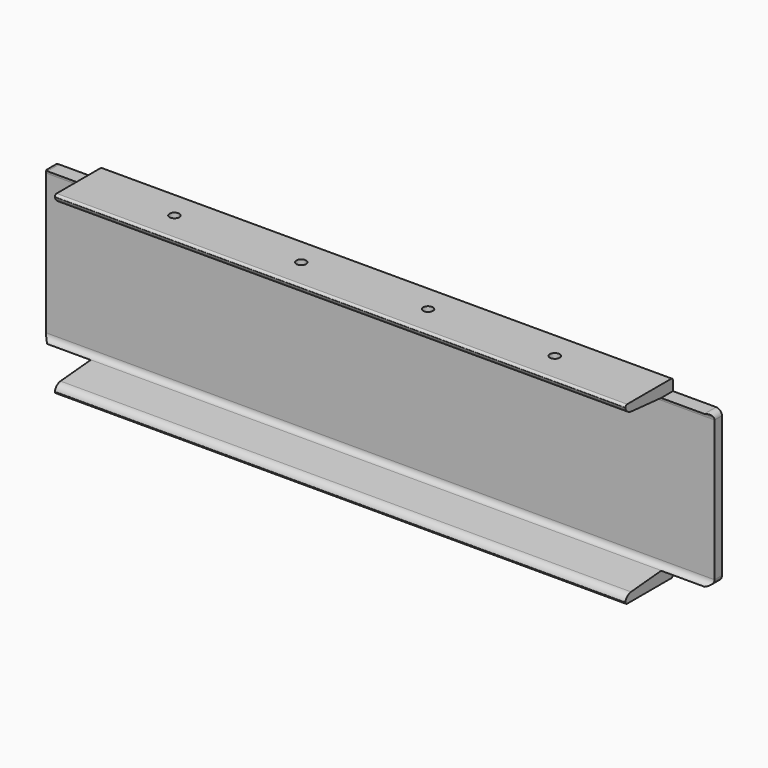
from build123d import *

# Parameters (mm, degrees)
F1_DEPTH    = 290
F2_T1_DEPTH = 611.1034588044
F3_R        = 4.25
F4_DEPTH    = 25
F5_W        = 60
F5_H        = 130.8605410159
F6_DEPTH    = 10.2
F7_R        = 5


# Not quite as in the source:
# - a fillet or chamfer that OpenCascade refuses, or shapes differently, is made with other operations: its cross-section is extruded or revolved along the edge and cut away or added
# - a pattern or mirror of a feature is missing from the dataset's text; its kind, count and spacing are read off the source's solid


with BuildPart() as f1:
    # F0 (on Right) → F1 (new body, symmetric)
    with BuildSketch(Plane.YZ):
        with BuildLine():
            ThreePointArc((-25.83, -74.2), (-25.2442135624, -75.6142135624), (-23.83, -76.2))
            Line((-23.83, -76.2), (23.83, -76.2))
            ThreePointArc((23.83, -76.2), (25.2442135624, -75.6142135624), (25.83, -74.2))
            Line((25.83, -74.2), (25.83, 74.2))
            ThreePointArc((25.83, 74.2), (25.2442135624, 75.6142135624), (23.83, 76.2))
            Line((23.83, 76.2), (-23.83, 76.2))
            ThreePointArc((-23.83, 76.2), (-25.2442135624, 75.6142135624), (-25.83, 74.2))
            Line((-25.83, 74.2), (-25.83, 69.4007524114))
            Line((-25.83, 69.4007524114), (13.2857787137, 65.978565209))
            ThreePointArc((13.2857787137, 65.978565209), (16.5363866841, 64.3755427566), (17.85, 60.9975917185))
            Line((17.85, 60.9975917185), (17.85, -60.9975917185))
            ThreePointArc((17.85, -60.9975917185), (16.5363866841, -64.3755427566), (13.2857787137, -65.978565209))
            Line((13.2857787137, -65.978565209), (-25.83, -69.4007524114))
            Line((-25.83, -69.4007524114), (-25.83, -74.2))
        make_face()
    extrude(amount=F1_DEPTH, both=True)

    # F2: fillet of radius 7 on 2 edges, made by hand

    # F2_s2 → F2_t1 (cut)
    with BuildSketch(Plane.YZ.offset(-305.5517294022)):
        with BuildLine():
            ThreePointArc((-25.83, -74.2), (-23.5930536317, -70.5297202282), (-19.6329798493, -68.8585834006))
            Line((-19.6329798493, -68.8585834006), (-19.6451816533, -68.7191161428))
            Line((-19.6451816533, -68.7191161428), (-25.842201804, -69.2612851537))
            Line((-25.842201804, -69.2612851537), (-25.97, -69.4007524114))
            ThreePointArc((-25.97, -69.4007524114), (-25.97, -71.8003762057), (-25.966142207, -74.1673610743))
            Line((-25.966142207, -74.1673610743), (-25.83, -74.2))
        make_face()
        with BuildLine():
            ThreePointArc((-19.6329798493, 68.8585834006), (-23.5930536317, 70.5297202282), (-25.83, 74.2))
            Line((-25.83, 74.2), (-25.966142207, 74.1673610743))
            ThreePointArc((-25.966142207, 74.1673610743), (-25.97, 71.8003762057), (-25.97, 69.4007524114))
            Line((-25.97, 69.4007524114), (-25.842201804, 69.2612851537))
            Line((-25.842201804, 69.2612851537), (-19.6451816533, 68.7191161428))
            Line((-19.6451816533, 68.7191161428), (-19.6329798493, 68.8585834006))
        make_face()
    extrude(amount=F2_T1_DEPTH, mode=Mode.SUBTRACT)

    # F3 (on face) → F4 (cut)
    with BuildSketch(Plane.XY.offset(76.2)):
        with Locations((-275, 0.83)):
            Circle(F3_R)
        with Locations((-165, 0.83)):
            Circle(F3_R)
        with Locations((-55, 0.83)):
            Circle(F3_R)
        with Locations((55, 0.83)):
            Circle(F3_R)
        with Locations((165, 0.83)):
            Circle(F3_R)
        with Locations((275, 0.83)):
            Circle(F3_R)
    extrude(amount=-F4_DEPTH, mode=Mode.SUBTRACT)

    # F5 (on face) → F6 (cut)
    with BuildSketch(Plane.XY.offset(76.2)):
        with Locations((-277.5, 8.7228175253)):
            Rectangle(F5_W, F5_H)
        with Locations((277.5, 8.7228175253)):
            Rectangle(F5_W, F5_H)
    f6 = extrude(amount=-F6_DEPTH, mode=Mode.SUBTRACT)

    # F6_copies: F6 across plane
    add(f6.mirror(Plane(origin=(0, 0, 0), x_dir=(-1, 0, 0), z_dir=(0, 0, -1))), mode=Mode.SUBTRACT)

    # F7
    f7_edges = [f1.edges().sort_by_distance(p)[0] for p in [
        (-290, 19.435389, 66),
        (290, 19.435389, 66),
        (290, 19.435389, -66),
        (-290, 19.435389, -66),
    ]]
    fillet(f7_edges, radius=F7_R)


solid = f1.part
